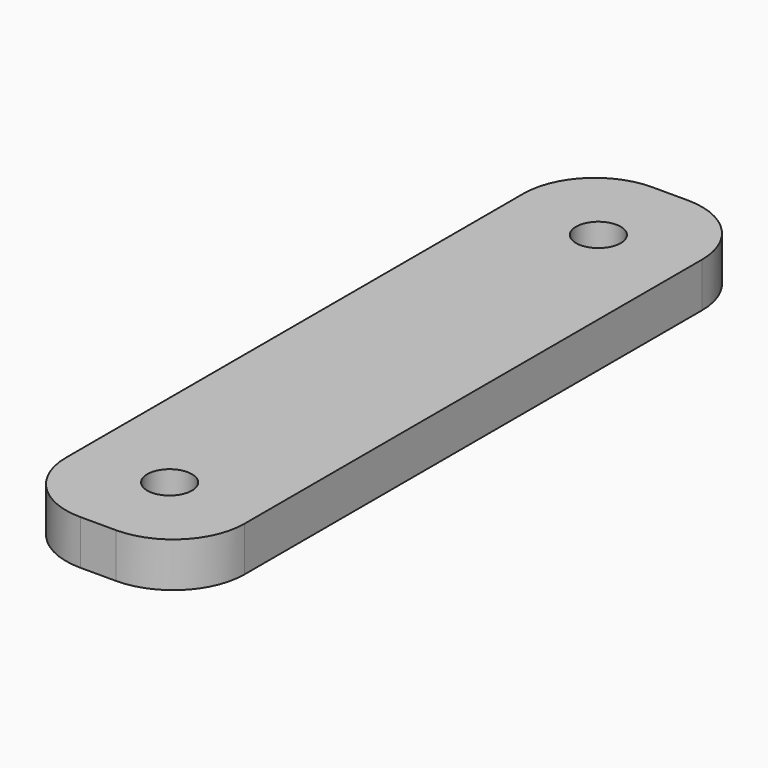
from build123d import *

# Parameters (mm, degrees)
F0_W     = 12.7
F0_H     = 50.8
F0_R     = 1.5875
F1_DEPTH = 3.175
F2_R     = 5.08


# Not quite as in the source:
# - a length typed as a fraction of an inch, garbled in the dataset ("3 / 203.2 mm" for 3/8 in), is restored


with BuildPart() as f1:
    # F0 (on Top) → F1 (new body)
    with BuildSketch(Plane.XY):
        with Locations((6.35, 25.4)):
            Rectangle(F0_W, F0_H)
        with Locations((6.35, 6.35)):
            Circle(F0_R, mode=Mode.SUBTRACT)
        with Locations((6.35, 44.45)):
            Circle(F0_R, mode=Mode.SUBTRACT)
    extrude(amount=F1_DEPTH)

    # F2
    f2_edges = [f1.edges().sort_by_distance(p)[0] for p in [
        (12.7, 0, 1.5875),
        (0, 0, 1.5875),
        (12.7, 50.8, 1.5875),
        (0, 50.8, 1.5875),
    ]]
    fillet(f2_edges, radius=F2_R)


solid = f1.part
